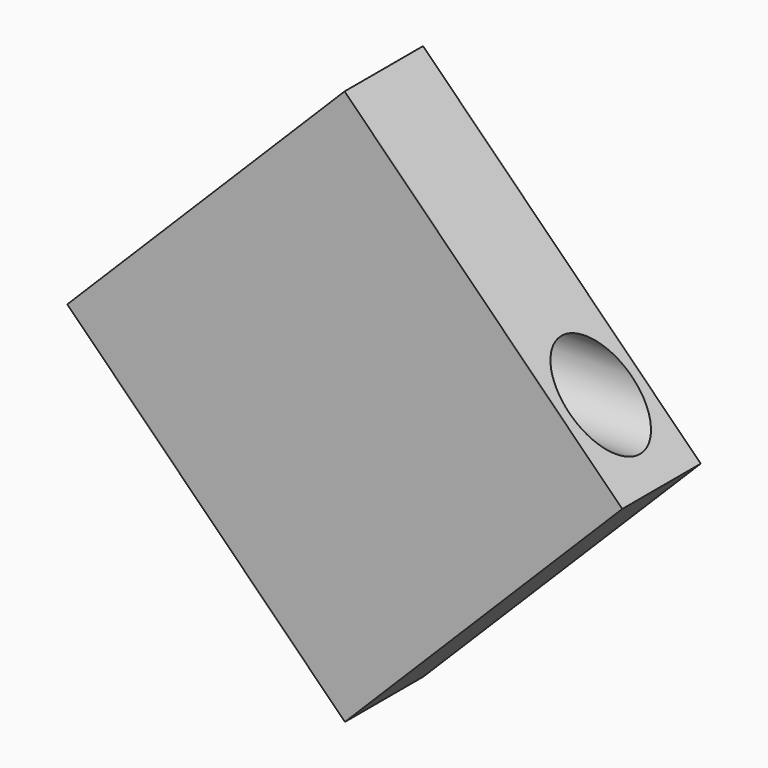
from build123d import *

# Parameters (mm, degrees)
F0_W      = 203.2
F0_H      = 44.45
F1_DEPTH  = 3.175
F3_DEPTH  = 6.35
F5_DEPTH  = 25.4
F6_DEPTH  = 25.4
F8_DEPTH  = 12.7
F9_R      = 5.08
F10_DEPTH = 76.2
F12_DEPTH = 25.4


with BuildPart() as f1:
    # F0 (on Front) → F1 (new body, symmetric)
    with BuildSketch(Plane.XZ):
        with Locations((2.1883048997, 22.225)):
            Rectangle(F0_W, F0_H)
    extrude(amount=F1_DEPTH, both=True)

    # F2 (on face) → F3 (join, symmetric)
    with BuildSketch(Plane.XZ.offset(3.175)):
        Polygon((2.2116978689, -13.6960168671), (38.1093217669, 22.2483929692), (2.1649119306, 58.1460168671), (-33.7327119674, 22.2016070308), align=None)
    extrude(amount=F3_DEPTH, both=True)


with BuildPart() as f1_1:
    # F4: moved
    add(f1.part.moved(Location((-2.20971, 0, 0))))

    # F5 (cut): a face of the model
    f5_faces = [f1_1.faces().sort_by_distance(p)[0] for p in [
        (-62.9576531363, -3.175, 22.225592552),
    ]]
    extrude(f5_faces, amount=-F5_DEPTH, mode=Mode.SUBTRACT)

    # F6 (cut): a face of the model
    f6_faces = [f1_1.faces().sort_by_distance(p)[0] for p in [
        (62.9148429358, -3.175, 22.224407448),
    ]]
    extrude(f6_faces, amount=-F6_DEPTH, mode=Mode.SUBTRACT)

    # F7 (on face) → F8 (join)
    with BuildSketch(Plane.XZ.offset(9.525)):
        Polygon((35.8996117669, 58.1460168671), (-0.0447980694, 58.1460168671), (35.8996117669, 22.2483929692), align=None)
        Polygon((-35.9424219674, 22.2016070308), (-0.0447980694, 58.1460168671), (-35.9424219674, 58.1460168671), align=None)
    extrude(amount=-F8_DEPTH)

    # F9 (on face) → F10 (cut)
    with BuildSketch(Plane.YZ.offset(35.8996117669)):
        with Locations((-3.175, 30.1041658968)):
            Circle(F9_R)
    extrude(amount=-F10_DEPTH, mode=Mode.SUBTRACT)

    # F11 (on face) → F12 (cut)
    with BuildSketch(Plane.XZ.offset(9.525)):
        Polygon((35.8996117669, 58.1460168671), (-0.0447980694, 58.1460168671), (35.8996117669, 22.2483929692), align=None)
        Polygon((-35.9424219674, 58.1460168671), (-35.9424219674, 22.2016070308), (-0.0447980694, 58.1460168671), align=None)
    extrude(amount=-F12_DEPTH, mode=Mode.SUBTRACT)


solid = f1_1.part
